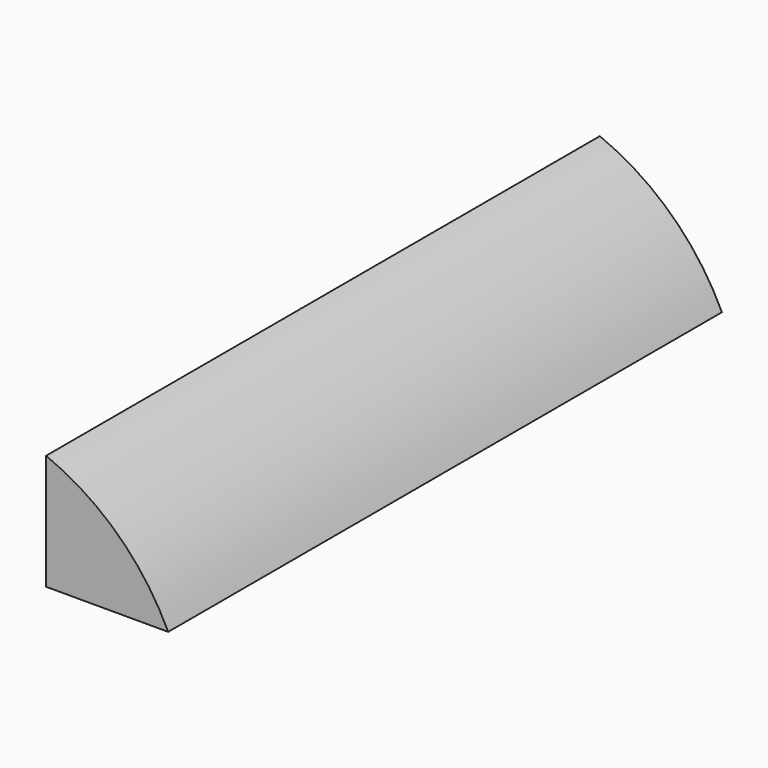
from build123d import *

# Parameters (mm, degrees)
F0_W        = 6.25
F0_H        = 30
F1_DEPTH    = 5
F2_T1_DEPTH = 76.3512405443


# Not quite as in the source:
# - a fillet or chamfer that OpenCascade refuses, or shapes differently, is made with other operations: its cross-section is extruded or revolved along the edge and cut away or added


with BuildPart() as f1:
    # F0 (on Top) → F1 (new body)
    with BuildSketch(Plane.XY):
        Rectangle(F0_W, F0_H)
    extrude(amount=F1_DEPTH)

    # F2: fillet of radius 10 on 1 edges, made by hand

    # F2_s2 → F2_t1 (cut)
    with BuildSketch(Plane.XZ.offset(-38.1756202722)):
        with BuildLine():
            ThreePointArc((3.125, -4.2702481089), (1.4165619759, 1.3199218349), (-3.125, 5))
            Line((-3.125, 5), (-3.05, 5.1854049622))
            ThreePointArc((-3.05, 5.1854049622), (0, 5.2), (3.125, 5.2))
            Line((3.125, 5.2), (3.325, 5))
            Line((3.325, 5), (3.325, -4.2702481089))
            Line((3.325, -4.2702481089), (3.125, -4.2702481089))
        make_face()
    extrude(amount=F2_T1_DEPTH, mode=Mode.SUBTRACT)


solid = f1.part
